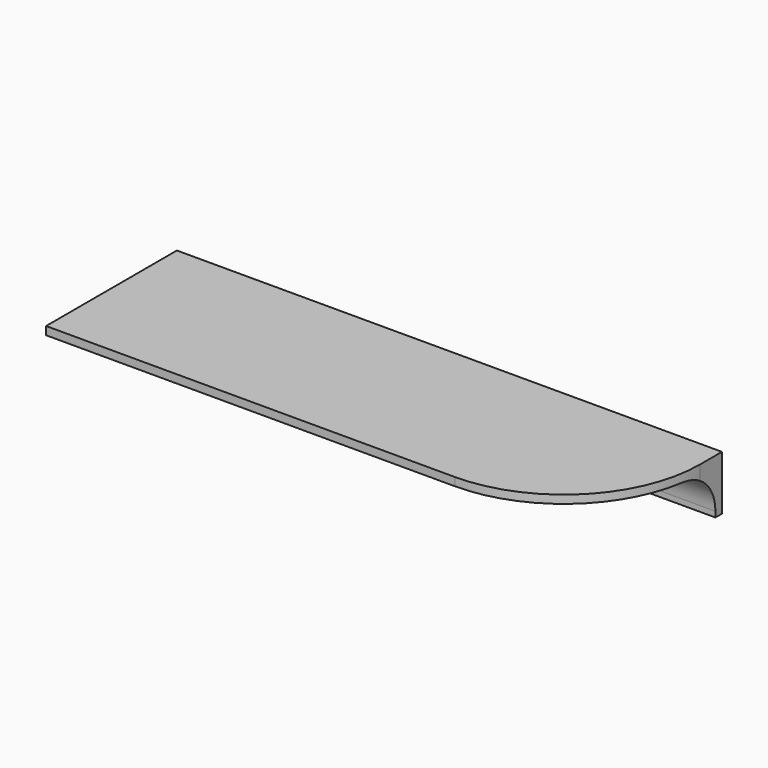
from build123d import *

# Parameters (mm, degrees)
F1_DEPTH = 3
F2_W     = 200
F2_H     = 17
F3_DEPTH = 3
F4_R     = 15


with BuildPart() as f1:
    # F0 (on Top) → F1 (new body)
    with BuildSketch(Plane.XY):
        with BuildLine():
            Line((91.016510874, -5.0278047089), (-108.983489126, -5.0278047089))
            Line((-108.983489126, -5.0278047089), (-108.983489126, -65.0278047089))
            Line((-108.983489126, -65.0278047089), (41.016510874, -65.0278047089))
            ThreePointArc((41.016510874, -65.0278047089), (76.3718499334, -50.3831437682), (91.016510874, -15.0278047089))
            Line((91.016510874, -15.0278047089), (91.016510874, -5.0278047089))
        make_face()
    extrude(amount=F1_DEPTH)

    # F2 (on face) → F3 (join)
    with BuildSketch(Plane(origin=(0, -5.0278047089, 0), x_dir=(-1, 0, 0), z_dir=(0, 1, 0))):
        with Locations((8.983489126, -8.5)):
            Rectangle(F2_W, F2_H)
    extrude(amount=-F3_DEPTH)

    # F4
    f4_edges = [f1.edges().sort_by_distance(p)[0] for p in [
        (-8.983489, -8.027805, 0),
    ]]
    fillet(f4_edges, radius=F4_R)


solid = f1.part
